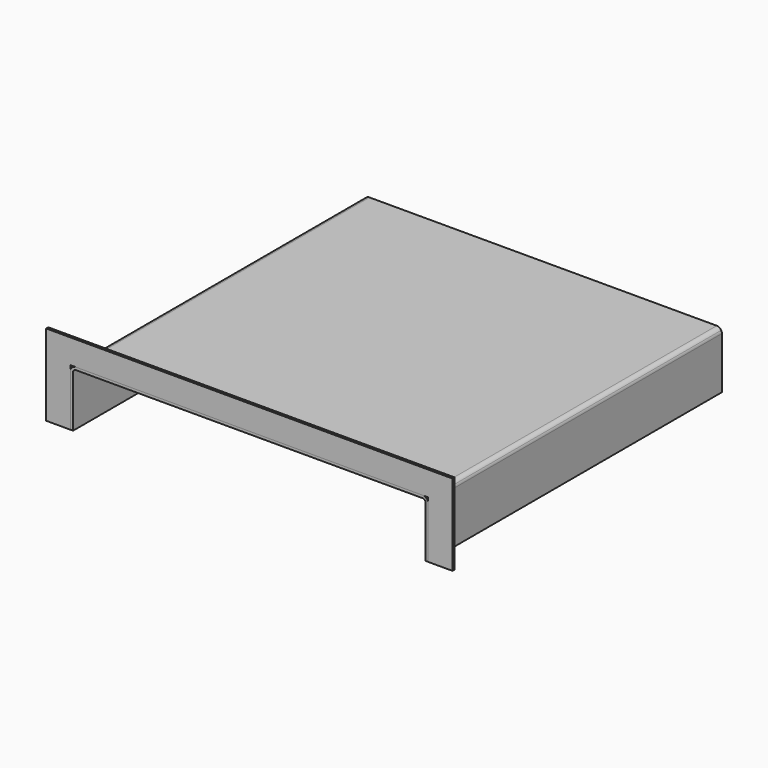
from build123d import *

# Parameters (mm, degrees)
F1_DEPTH = 1.6
F2_DEPTH = 226


# Not quite as in the source:
# - ends of sketch curves that miss each other by under 0.0002 mm in the source are joined


with BuildPart() as f1:
    # F0 (on Front) → F1 (new body)
    with BuildSketch(Plane.XZ):
        Polygon((-105.330753, 62.095962), (-325.330753, 62.095962), (-325.330753, 47.095962), (-322.130753, 47.095962), (-108.530753, 47.095962), (-105.330753, 47.095962), align=None)
        Polygon((-90.330753, 62.095962), (-105.330753, 62.095962), (-105.330753, 47.095962), (-105.330753, 45.495962), (-105.330753, 43.895962), (-105.330753, 12.095962), (-90.330753, 12.095962), align=None)
        Polygon((-325.330753, 47.095962), (-325.330753, 62.095962), (-340.330753, 62.095962), (-340.330753, 12.095962), (-325.330753, 12.095962), (-325.330753, 43.895962), (-325.330753, 45.495962), align=None)
    extrude(amount=-F1_DEPTH)


with BuildPart() as f2:
    # F0 (on Front) → F2 (new body)
    with BuildSketch(Plane.XZ):
        with BuildLine():
            ThreePointArc((-105.330753, 43.895962), (-105.4397903748, 44.7241830149), (-105.7594717809, 45.4959621265))
            Line((-105.7594717809, 45.4959621265), (-108.530753, 45.495962))
            ThreePointArc((-108.530753, 45.495962), (-107.3993821501, 45.0273328499), (-106.930753, 43.895962))
            Line((-106.930753, 43.895962), (-106.930753, 12.095962))
            Line((-106.930753, 12.095962), (-105.330753, 12.095962))
            Line((-105.330753, 12.095962), (-105.330753, 43.895962))
        make_face()
        with BuildLine():
            Line((-108.530753, 47.095962), (-322.130753, 47.095962))
            ThreePointArc((-322.130753, 47.095962), (-323.7307529368, 46.6672433286), (-324.9020342191, 45.4959621265))
            Line((-324.9020342191, 45.4959621265), (-322.130753, 45.495962))
            Line((-322.130753, 45.495962), (-108.530753, 45.495962))
            Line((-108.530753, 45.495962), (-105.7594717809, 45.495962))
            ThreePointArc((-105.7594717809, 45.495962), (-106.9307530632, 46.6672433286), (-108.530753, 47.095962))
        make_face()
        with BuildLine():
            ThreePointArc((-324.9020342191, 45.4959621265), (-325.2217156252, 44.7241830149), (-325.330753, 43.895962))
            Line((-325.330753, 43.895962), (-325.330753, 12.095962))
            Line((-325.330753, 12.095962), (-323.730753, 12.095962))
            Line((-323.730753, 12.095962), (-323.730753, 43.895962))
            ThreePointArc((-323.730753, 43.895962), (-323.2621238499, 45.0273328499), (-322.130753, 45.495962))
            Line((-322.130753, 45.495962), (-324.9020342191, 45.4959621265))
        make_face()
    extrude(amount=-F2_DEPTH)


solid = Compound([f1.part, f2.part])
